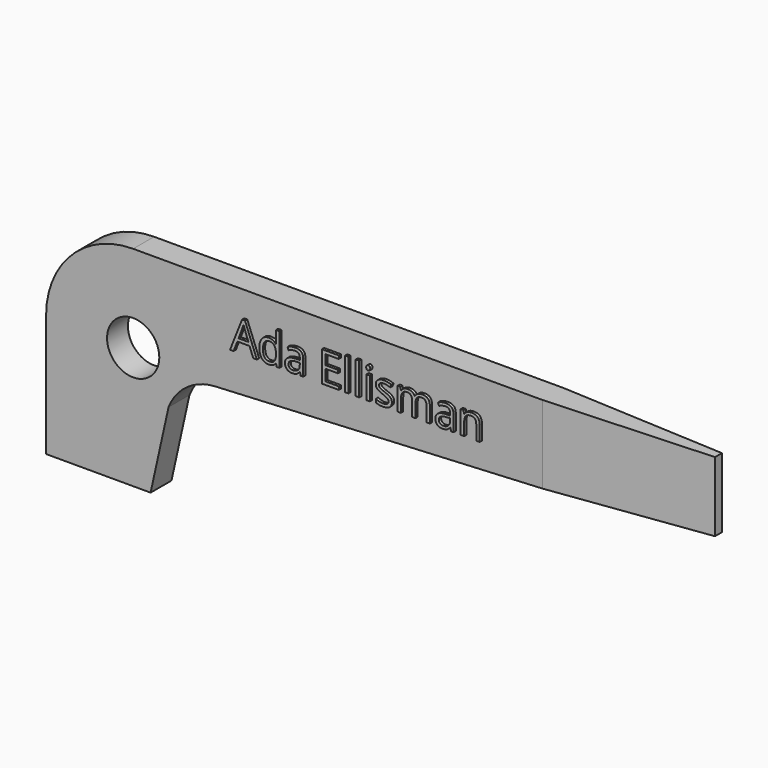
from build123d import *

# Parameters (mm, degrees)
F1_DEPTH     = 2.38125
F2_R         = 2.38125
F3_DEPTH     = 25.4
F5_DEPTH     = 25.4
F6_TEXT_SIZE = 3.8739461969
F7_DEPTH     = 0.254


# Not quite as in the source:
# - Text() gives the source's letters only with a copy of the font that has no kerning and outlines rounded to 1/6400 em; it was checked with that copy


with BuildPart() as f1:
    # F0 (on Front) → F1 (new body)
    with BuildSketch(Plane.XZ):
        with BuildLine():
            Line((60.325, 19.05), (7.9375, 19.05))
            ThreePointArc((7.9375, 19.05), (2.3248399243, 16.7251600757), (0, 11.1125))
            Line((0, 11.1125), (0, 0))
            Line((0, 0), (9.525, 0))
            Line((9.525, 0), (11.1604742097, 7.3929509647))
            ThreePointArc((11.1604742097, 7.3929509647), (12.8362796751, 9.5409555175), (15.4080715284, 10.4399183532))
            Line((15.4080715284, 10.4399183532), (60.325, 12.7))
            Line((60.325, 12.7), (60.325, 19.05))
        make_face()
    extrude(amount=F1_DEPTH)

    # F2 (on face) → F3 (cut)
    with BuildSketch(Plane.XZ.offset(2.38125)):
        with Locations((7.9375, 11.1125)):
            Circle(F2_R)
    extrude(amount=-F3_DEPTH, mode=Mode.SUBTRACT)

    # F4 (on face) → F5 (cut)
    with BuildSketch(Plane.XY.offset(19.05)):
        Polygon((60.325, -2.38125), (60.325, -1.5875), (45.24375, -2.38125), align=None)
        Polygon((45.24375, 0), (60.325, -0.79375), (60.325, 0), align=None)
    extrude(amount=-F5_DEPTH, mode=Mode.SUBTRACT)

    # F6 (on face) → F7 (join)
    with BuildSketch(Plane.XZ.offset(2.38125)):
        with Locations((16.9706270099, 13.990025036)):
            Text('Ada Ellisman', F6_TEXT_SIZE, font='Open Sans', text_align=(TextAlign.LEFT, TextAlign.BOTTOM))
    extrude(amount=F7_DEPTH)


solid = f1.part
